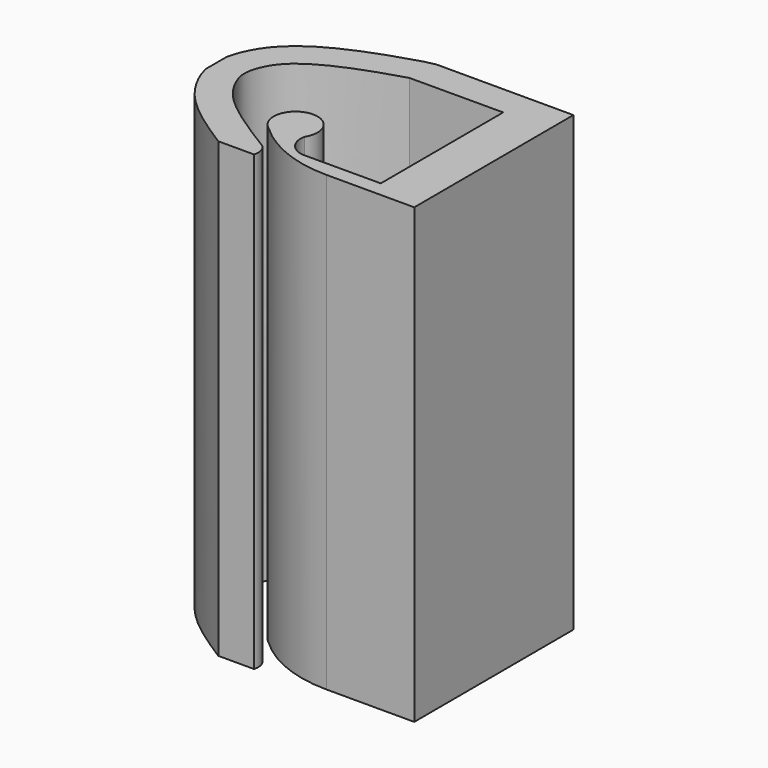
from build123d import *

# Parameters (mm, degrees)
F1_DEPTH = 112.014


# Not quite as in the source:
# - the dataset's text gives a spline's control points without its knots; the knots are read off the source's solid


with BuildPart() as f1:
    # F0 (on Top) → F1 (new body)
    with BuildSketch(Plane.XY):
        with BuildLine():
            add(Edge.make_bspline(
                [(-3.6331126697, 24.2653177011), (-5.0309529603, 23.8382389404), (-7.8975267056, 22.9629912291), (-11.718090926, 21.6763315248), (-14.5334664534, 20.6006395255), (-16.182496931, 19.9268284227), (-17.8704875446, 19.2041676976), (-20.0294844318, 18.2054412077), (-22.2037087742, 17.0613993179), (-23.9249386903, 16.039932435), (-25.2004920279, 15.2133999646), (-26.4542240511, 14.3172946942), (-27.4750075017, 13.5025428385), (-28.2728766175, 12.8021712395), (-28.8604532589, 12.2502355378), (-29.4356650634, 11.6692589018), (-30.1827509214, 10.8516299584), (-31.0239328159, 9.8088760785), (-31.9008477948, 8.5318465415), (-32.6494845802, 7.2464120404), (-33.2785601353, 5.9641415612), (-33.7960973203, 4.6948725196), (-34.2100695572, 3.4449745693), (-34.4363698162, 2.5702966484), (-34.5371913675, 2.1084842073), (-34.5492400229, 2.0520120912)],
                knots=[0, 0, 0, 0, 0.0625, 0.125, 0.15625, 0.171875, 0.1875, 0.21875, 0.25, 0.265625, 0.28125, 0.296875, 0.3125, 0.3203125, 0.328125, 0.3359375, 0.34375, 0.359375, 0.375, 0.390625, 0.40625, 0.421875, 0.4375, 0.453125, 0.4553050227, 0.4553050227, 0.4553050227, 0.4553050227], degree=3))
            Line((-34.5492400229, 2.0520120912), (-34.5492400229, -4.4208203143))
            add(Edge.make_bspline(
                [(-34.5492400229, -4.4208203143), (-34.489113708, -4.6837345013), (-34.3746747946, -5.1291131913), (-34.1945112231, -5.731759966), (-33.9668488949, -6.420929735), (-33.642322086, -7.288220263), (-33.1904909143, -8.3348803349), (-32.6737742662, -9.3918843822), (-32.0900994525, -10.4577631597), (-31.43685187, -11.53009527), (-30.7114207375, -12.60472958), (-30.0440150101, -13.4982936399), (-29.4716351251, -14.2082014467), (-28.8705883228, -14.9162187281), (-28.0970743584, -15.7613933068), (-27.1403248028, -16.7214580423), (-26.1610852679, -17.6338632647), (-24.8327091865, -18.7942102065), (-23.1425198927, -20.1505242113), (-21.4473806936, -21.4011499112), (-20.1095106505, -22.3449978474), (-19.1227149693, -23.0242265175), (-18.1519831057, -23.6798380791), (-16.8678427909, -24.5320372769), (-15.4062427324, -25.4786943537), (-14.2798180934, -26.1918329815), (-13.7791677315, -26.5064007463)],
                knots=[0.5363355239, 0.5363355239, 0.5363355239, 0.5363355239, 0.546875, 0.5546875, 0.5625, 0.578125, 0.59375, 0.609375, 0.625, 0.640625, 0.65625, 0.671875, 0.6796875, 0.6875, 0.703125, 0.71875, 0.734375, 0.75, 0.78125, 0.8125, 0.828125, 0.84375, 0.859375, 0.875, 0.90625, 0.931578944, 0.931578944, 0.931578944, 0.931578944], degree=3))
            Line((-13.7791677315, -26.5064007463), (-4.9322219839, -26.5064007463))
            ThreePointArc((-4.9322219839, -26.5064007463), (-4.8975988419, -24.462141672), (-5.9359231964, -22.7008704096))
            add(Edge.make_bspline(
                [(-1.4808116248, 17.2207783908), (-5.1765813608, 16.0916188086), (-12.758111735, 13.7752521836), (-24.9027070765, 7.6414710987), (-27.8190436978, 0.1217712147), (-27.3803734584, -3.8196436866), (-23.9090668472, -10.4750472767), (-14.9292775561, -17.1682110986), (-8.9073592794, -20.8728602085), (-5.9359231964, -22.7008704096)],
                knots=[0, 0, 0, 0, 0.1652446349, 0.3389841111, 0.4667292372, 0.558017353, 0.684380504, 0.844261726, 1, 1, 1, 1], degree=3))
            Line((-1.4808116248, 17.2207783908), (21.6409831651, 17.2708898329))
            Line((21.6409831651, 17.2708898329), (21.723201308, -20.6651771691))
            Line((21.723201308, -20.6651771691), (2.4085581355, -20.7070374413))
            ThreePointArc((2.4085581355, -20.7070374413), (0.366288536, -19.9926081592), (-1.1964672012, -18.4962563217))
            ThreePointArc((-1.1964672012, -18.4962563217), (-1.9597863377, -16.6342281191), (-1.9197666552, -14.6222133189))
            ThreePointArc((-1.9197666552, -14.6222133189), (-7.5485703286, -6.3942683653), (-9.6057578921, -16.1487795413))
            ThreePointArc((-9.6057578921, -16.1487795413), (0.0367461623, -22.2913896471), (11.2658366561, -24.4401264936))
            Line((11.2658366561, -24.4401264936), (33.024482429, -24.4401264936))
            Line((33.024482429, -24.4401264936), (32.9176075757, 24.8727314174))
            Line((32.9176075757, 24.8727314174), (-0.8711330011, 24.8727314174))
            Line((-0.8711330011, 24.8727314174), (-3.6331126697, 24.2653177011))
        make_face()
    extrude(amount=-F1_DEPTH)


solid = f1.part
